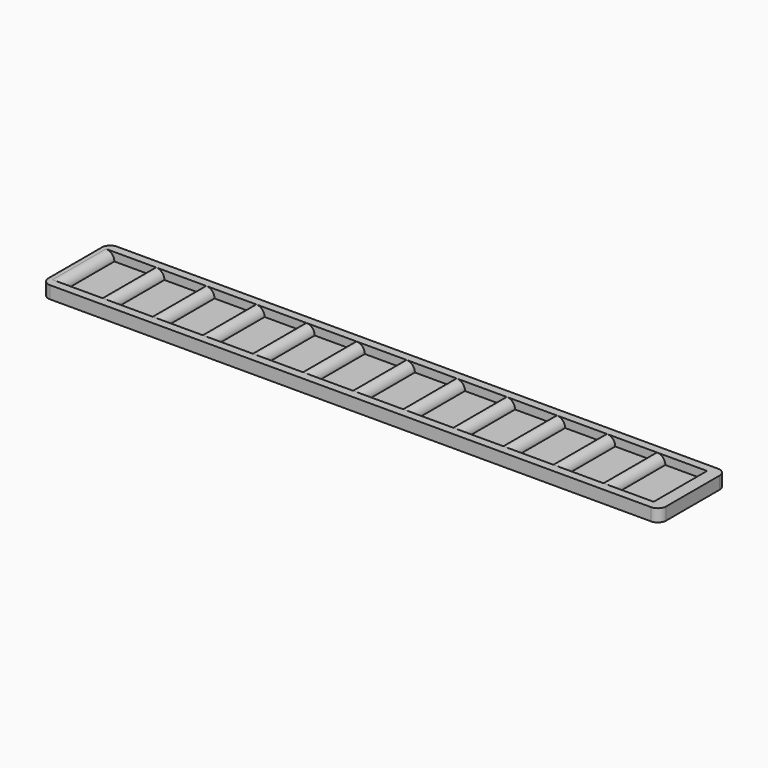
from build123d import *

# Parameters (mm, degrees)
F0_W     = 148
F0_H     = 20
F1_DEPTH = 3
F2_W     = 10
F2_H     = 16
F3_DEPTH = 2
F4_R     = 2
F4_R_2   = 1.99999


# Not quite as in the source:
# - a fillet or chamfer is up to 0.001 mm smaller than in the source, because OpenCascade refuses the exact size


with BuildPart() as f1:
    # F0 (on Top) → F1 (new body)
    with BuildSketch(Plane.XY):
        with Locations((-1.0154450944, 0.4536062479)):
            Rectangle(F0_W, F0_H)
    extrude(amount=F1_DEPTH)

    # F2 (on face) → F3 (cut)
    with BuildSketch(Plane.XY.offset(3)):
        with Locations((-67.0154450944, 0.4536062479)):
            Rectangle(F2_W, F2_H)
        with Locations((-55.0154450944, 0.4536062479)):
            Rectangle(F2_W, F2_H)
        with Locations((-43.0154450944, 0.4536062479)):
            Rectangle(F2_W, F2_H)
        with Locations((-31.0154450944, 0.4536062479)):
            Rectangle(F2_W, F2_H)
        with Locations((-19.0154450944, 0.4536062479)):
            Rectangle(F2_W, F2_H)
        with Locations((-7.0154450944, 0.4536062479)):
            Rectangle(F2_W, F2_H)
        with Locations((4.9845549056, 0.4536062479)):
            Rectangle(F2_W, F2_H)
        with Locations((16.9845549056, 0.4536062479)):
            Rectangle(F2_W, F2_H)
        with Locations((28.9845549056, 0.4536062479)):
            Rectangle(F2_W, F2_H)
        with Locations((40.9845549056, 0.4536062479)):
            Rectangle(F2_W, F2_H)
        with Locations((52.9845549056, 0.4536062479)):
            Rectangle(F2_W, F2_H)
        with Locations((64.9845549056, 0.4536062479)):
            Rectangle(F2_W, F2_H)
    extrude(amount=-F3_DEPTH, mode=Mode.SUBTRACT)

    # F4 (call 1 of 16: OpenCascade refuses the feature's edges together)
    f4_edges = [f1.edges().sort_by_distance(p)[0] for p in [
        (-75.015445, -9.546394, 1.5),
    ]]
    fillet(f4_edges, radius=F4_R)

    # F4#2 (call 2 of 16)
    f4_2_edges = [f1.edges().sort_by_distance(p)[0] for p in [
        (72.984555, -9.546394, 1.5),
    ]]
    fillet(f4_2_edges, radius=F4_R)

    # F4#3 (call 3 of 16)
    f4_3_edges = [f1.edges().sort_by_distance(p)[0] for p in [
        (72.984555, 10.453606, 1.5),
    ]]
    fillet(f4_3_edges, radius=F4_R)

    # F4#4 (call 4 of 16)
    f4_4_edges = [f1.edges().sort_by_distance(p)[0] for p in [
        (-75.015445, 10.453606, 1.5),
    ]]
    fillet(f4_4_edges, radius=F4_R)

    # F4#5 (call 5 of 16) (radius 2 in the source; OpenCascade refuses exactly that, so slightly less here)
    f4_5_edges = [f1.edges().sort_by_distance(p)[0] for p in [
        (-72.015445, 0.453606, 3),
    ]]
    fillet(f4_5_edges, radius=F4_R_2)

    # F4#6 (call 6 of 16) (radius 2 in the source; OpenCascade refuses exactly that, so slightly less here)
    f4_6_edges = [f1.edges().sort_by_distance(p)[0] for p in [
        (-60.015445, 0.453606, 3),
    ]]
    fillet(f4_6_edges, radius=F4_R_2)

    # F4#7 (call 7 of 16) (radius 2 in the source; OpenCascade refuses exactly that, so slightly less here)
    f4_7_edges = [f1.edges().sort_by_distance(p)[0] for p in [
        (-48.015445, 0.453606, 3),
    ]]
    fillet(f4_7_edges, radius=F4_R_2)

    # F4#8 (call 8 of 16) (radius 2 in the source; OpenCascade refuses exactly that, so slightly less here)
    f4_8_edges = [f1.edges().sort_by_distance(p)[0] for p in [
        (-36.015445, 0.453606, 3),
    ]]
    fillet(f4_8_edges, radius=F4_R_2)

    # F4#9 (call 9 of 16) (radius 2 in the source; OpenCascade refuses exactly that, so slightly less here)
    f4_9_edges = [f1.edges().sort_by_distance(p)[0] for p in [
        (-24.015445, 0.453606, 3),
    ]]
    fillet(f4_9_edges, radius=F4_R_2)

    # F4#10 (call 10 of 16) (radius 2 in the source; OpenCascade refuses exactly that, so slightly less here)
    f4_10_edges = [f1.edges().sort_by_distance(p)[0] for p in [
        (-12.015445, 0.453606, 3),
    ]]
    fillet(f4_10_edges, radius=F4_R_2)

    # F4#11 (call 11 of 16) (radius 2 in the source; OpenCascade refuses exactly that, so slightly less here)
    f4_11_edges = [f1.edges().sort_by_distance(p)[0] for p in [
        (-0.015445, 0.453606, 3),
    ]]
    fillet(f4_11_edges, radius=F4_R_2)

    # F4#12 (call 12 of 16) (radius 2 in the source; OpenCascade refuses exactly that, so slightly less here)
    f4_12_edges = [f1.edges().sort_by_distance(p)[0] for p in [
        (11.984555, 0.453606, 3),
    ]]
    fillet(f4_12_edges, radius=F4_R_2)

    # F4#13 (call 13 of 16) (radius 2 in the source; OpenCascade refuses exactly that, so slightly less here)
    f4_13_edges = [f1.edges().sort_by_distance(p)[0] for p in [
        (23.984555, 0.453606, 3),
    ]]
    fillet(f4_13_edges, radius=F4_R_2)

    # F4#14 (call 14 of 16) (radius 2 in the source; OpenCascade refuses exactly that, so slightly less here)
    f4_14_edges = [f1.edges().sort_by_distance(p)[0] for p in [
        (35.984555, 0.453606, 3),
    ]]
    fillet(f4_14_edges, radius=F4_R_2)

    # F4#15 (call 15 of 16) (radius 2 in the source; OpenCascade refuses exactly that, so slightly less here)
    f4_15_edges = [f1.edges().sort_by_distance(p)[0] for p in [
        (47.984555, 0.453606, 3),
    ]]
    fillet(f4_15_edges, radius=F4_R_2)

    # F4#16 (call 16 of 16) (radius 2 in the source; OpenCascade refuses exactly that, so slightly less here)
    f4_16_edges = [f1.edges().sort_by_distance(p)[0] for p in [
        (59.984555, 0.453606, 3),
    ]]
    fillet(f4_16_edges, radius=F4_R_2)


solid = f1.part
